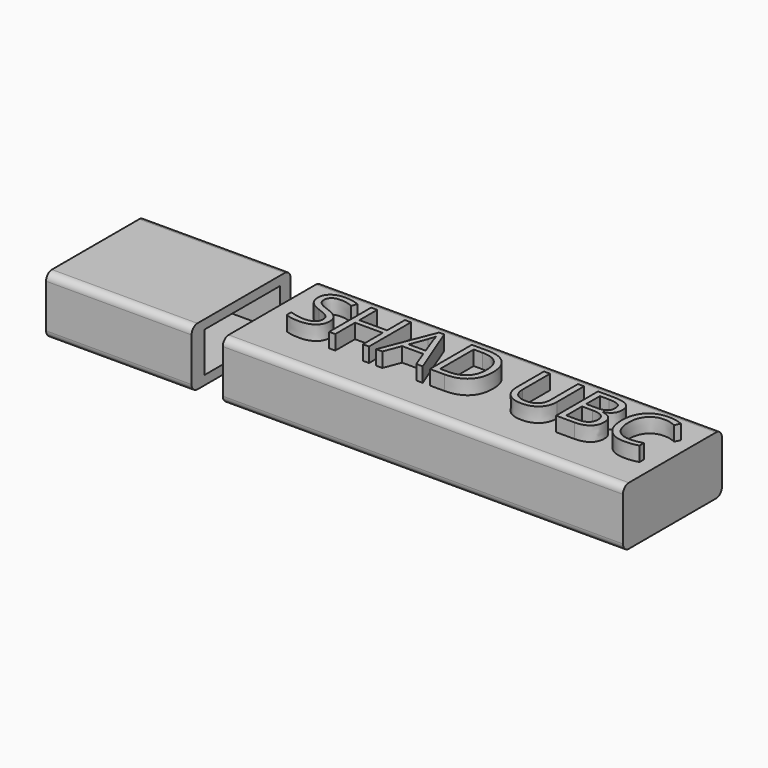
from build123d import *

# Parameters (mm, degrees)
F1_DEPTH     = 55
F3_W         = 12.4
F3_H         = 5
F4_DEPTH     = 14
F6_ANGLE     = 90
F5_TEXT_SIZE = 10.1003724512
F8_DEPTH     = 2
F10_DEPTH    = 20
F13_W        = 13
F13_H        = 5.5
F14_DEPTH    = 16


# Not quite as in the source:
# - Text() gives the source's letters only with a copy of the font that has no kerning and outlines rounded to 1/6400 em; it was checked with that copy


with BuildPart() as f1:
    # F0 (on Front) → F1 (new body)
    with BuildSketch(Plane.XZ):
        with BuildLine():
            ThreePointArc((8.5, 3), (8.2071067812, 3.7071067812), (7.5, 4))
            Line((7.5, 4), (-7.5, 4))
            ThreePointArc((-7.5, 4), (-8.2071067812, 3.7071067812), (-8.5, 3))
            Line((-8.5, 3), (-8.5, -3))
            ThreePointArc((-8.5, -3), (-8.2071067812, -3.7071067812), (-7.5, -4))
            Line((-7.5, -4), (7.5, -4))
            ThreePointArc((7.5, -4), (8.2071067812, -3.7071067812), (8.5, -3))
            Line((8.5, -3), (8.5, 3))
        make_face()
    extrude(amount=F1_DEPTH)


with BuildPart() as f1_1:
    # F2: moved
    add(f1.part.moved(Location((0, 27.4, 0))))

    # F3 (on face) → F4 (cut)
    with BuildSketch(Plane.XZ.offset(27.6)):
        Rectangle(F3_W, F3_H)
    extrude(amount=-F4_DEPTH, mode=Mode.SUBTRACT)


with BuildPart() as f1_2:
    # F6: moved
    add(f1_1.part.rotate(Axis((-8.5, 27.4, 0), (0, 0, -1)), F6_ANGLE))


with BuildPart() as f1_3:
    # F7: moved
    add(f1_2.part.moved(Location((37.7, -21.1, 0))))

    # F5 (on face) → F8 (join)
    with BuildSketch(Plane.XY.offset(4)):
        with Locations((-21.9588748653, -5.3973712146)):
            Text('SHAD UBC', F5_TEXT_SIZE, font='Open Sans', text_align=(TextAlign.LEFT, TextAlign.BOTTOM))
    extrude(amount=F8_DEPTH)


with BuildPart() as f10:
    # F9 (on Right) → F10 (new body)
    with BuildSketch(Plane.YZ):
        with BuildLine():
            Line((-13.5288010538, 8), (-28.5288010538, 8))
            ThreePointArc((-28.5288010538, 8), (-29.2359078349, 7.7071067812), (-29.5288010538, 7))
            Line((-29.5288010538, 7), (-29.5288010538, 1))
            ThreePointArc((-29.5288010538, 1), (-29.2359078349, 0.2928932188), (-28.5288010538, 0))
            Line((-28.5288010538, 0), (-13.5288010538, 0))
            ThreePointArc((-13.5288010538, 0), (-12.8216942726, 0.2928932188), (-12.5288010538, 1))
            Line((-12.5288010538, 1), (-12.5288010538, 7))
            ThreePointArc((-12.5288010538, 7), (-12.8216942726, 7.7071067812), (-13.5288010538, 8))
        make_face()
    extrude(amount=F10_DEPTH)


with BuildPart() as f10_1:
    # F11: moved
    add(f10.part.moved(Location((-53.2, 46.8, -4))))


with BuildPart() as f10_2:
    # F12: moved
    add(f10_1.part.moved(Location((104, -25.77, 0))))

    # F13 (on face) → F14 (cut)
    with BuildSketch(Plane.YZ.offset(70.8)):
        with Locations((0.2158132847, 0)):
            Rectangle(F13_W, F13_H)
    extrude(amount=-F14_DEPTH, mode=Mode.SUBTRACT)


with BuildPart() as f10_3:
    # F15: moved
    add(f10_2.part.moved(Location((-110, 0, 0))))


with BuildPart() as f1_4:
    # F16: moved
    add(f1_3.part.moved(Location((0, 2.19, 0))))


with BuildPart() as f10_4:
    # F17: moved
    add(f10_3.part.moved(Location((9.1, 0, 0))))


solid = Compound([f1_4.part, f10_4.part])
